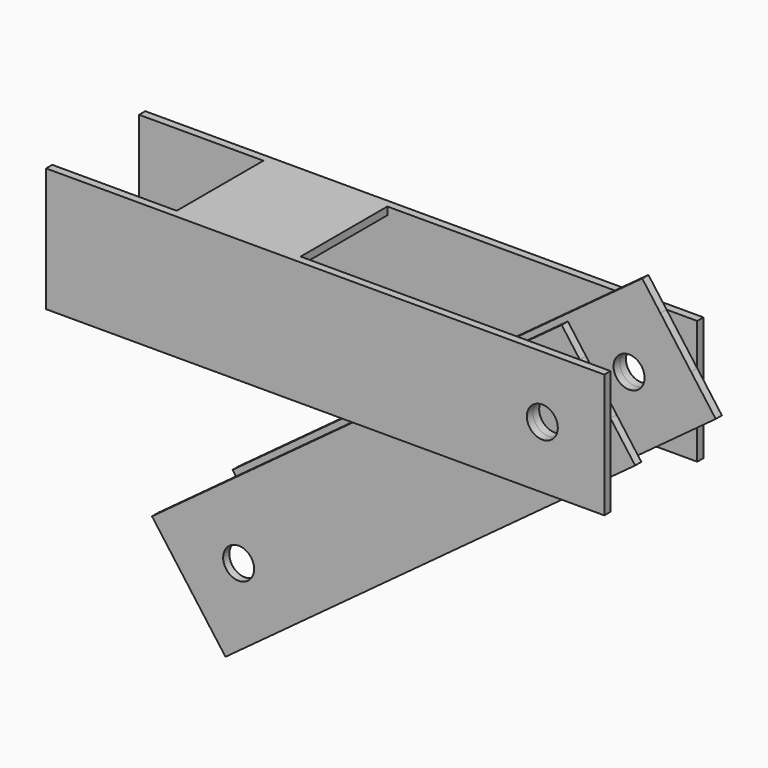
from build123d import *

# Parameters (mm, degrees)
F0_R     = 6.35
F1_DEPTH = 3.175
F0_W     = 50.8
F0_H     = 3.175
F2_DEPTH = 3.175
F5_DEPTH = 44.45


# Not quite as in the source:
# - a feature names something its author has since deleted; it is built from what else it names


with BuildPart() as f1:
    # F0 (on Front) → F1 (new body)
    with BuildSketch(Plane.XZ):
        Polygon((118.6567593262, 118.9230999827), (49.6727329072, 68.1230999827), (135.3432406738, 68.1230999827), (152.4, 80.6837378398), (152.4, 101.8663406565), (139.8393621429, 118.9230999827), align=None)
        with Locations((127, 93.5230999827)):
            Circle(F0_R, mode=Mode.SUBTRACT)
        Polygon((152.4, 101.8663406565), (152.4, 80.6837378398), (162.5141384166, 88.1318132601), align=None)
        Polygon((132.3912867226, 129.0372383994), (118.6567593262, 118.9230999827), (139.8393621429, 118.9230999827), align=None)
        Polygon((49.6727329072, 68.1230999827), (48.438574153, 67.214262561), (50.3212523839, 64.6576734898), (9.4158272446, 34.5348217958), (7.5331490138, 37.091410867), (-35.5141384166, 5.3912867226), (-5.3912867226, -35.5141384166), (135.3432406738, 68.1230999827), align=None)
        Circle(F0_R, mode=Mode.SUBTRACT)
        Polygon((50.3212523839, 64.6576734898), (48.438574153, 67.214262561), (7.5331490138, 37.091410867), (9.4158272446, 34.5348217958), align=None)
    extrude(amount=F1_DEPTH)


with BuildPart() as f2:
    # F0 (on Front) → F2 (new body)
    with BuildSketch(Plane.XZ):
        Polygon((-76.3788797785, 68.1230999827), (49.6727329072, 68.1230999827), (118.6567593262, 118.9230999827), (25.4, 118.9230999827), (25.4, 115.7480999827), (-25.4, 115.7480999827), (-25.4, 118.9230999827), (-76.3788797785, 118.9230999827), align=None)
        Polygon((118.6567593262, 118.9230999827), (49.6727329072, 68.1230999827), (135.3432406738, 68.1230999827), (152.4, 80.6837378398), (152.4, 101.8663406565), (139.8393621429, 118.9230999827), align=None)
        with Locations((127, 93.5230999827)):
            Circle(F0_R, mode=Mode.SUBTRACT)
        Polygon((152.4, 80.6837378398), (135.3432406738, 68.1230999827), (152.4, 68.1230999827), align=None)
        Polygon((152.4, 118.9230999827), (139.8393621429, 118.9230999827), (152.4, 101.8663406565), align=None)
        with Locations((0, 117.3355999827)):
            Rectangle(F0_W, F0_H)
    extrude(amount=-F2_DEPTH)


with BuildPart() as f4_1:
    # F4: instance of F1
    add(f1.part.mirror(Plane(origin=(63.5, -22.225, 46.7615499914), x_dir=(1, 0, 0), z_dir=(0, -1, 0))))


with BuildPart() as f4_2:
    # F4: instance of F2
    add(f2.part.mirror(Plane(origin=(63.5, -22.225, 46.7615499914), x_dir=(1, 0, 0), z_dir=(0, -1, 0))))


with BuildPart() as f2_1:
    add(f2.part)

    add(f4_2.part)  # F5 merges F4_2
    # F0 (on Front) → F5 (join, through all)
    with BuildSketch(Plane.XZ):
        with Locations((0, 117.3355999827)):
            Rectangle(F0_W, F0_H)
    extrude(amount=F5_DEPTH)


solid = Compound([f1.part, f4_1.part, f2_1.part])
